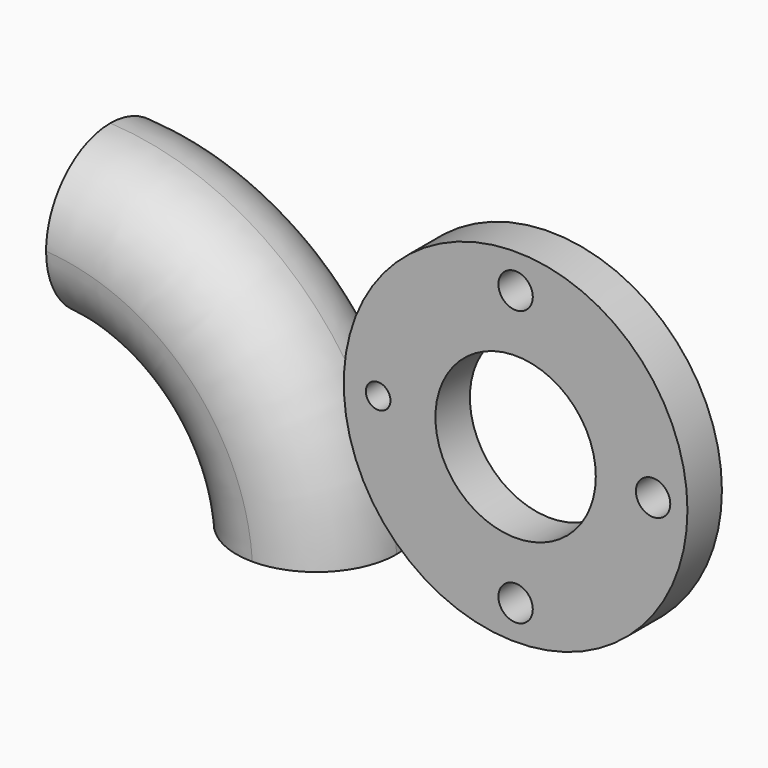
from build123d import *

# Parameters (mm, degrees)
F1_DEPTH    = 44.45
F2_T2_ANGLE = 160.6979741432
F2_T4_ANGLE = 241.2853924859
F2_T6_ANGLE = 160.6979741432
F2_T8_ANGLE = 241.2853924859
F3_R        = 95.25
F3_R_2      = 9.525
F3_R_3      = 6.8244070411
F3_R_4      = 44.45
F4_DEPTH    = 23.876


# Not quite as in the source:
# - a fillet or chamfer that OpenCascade refuses, or shapes differently, is made with other operations: its cross-section is extruded or revolved along the edge and cut away or added


with BuildPart() as f1:
    # F0 (on Front) → F1 (new body, symmetric)
    with BuildSketch(Plane.XZ):
        with BuildLine():
            Line((-141.7071309926, 88.9), (-141.7071309926, 0))
            ThreePointArc((-141.7071309926, 0), (-94.3529466908, -22.4958156982), (-71.8571309926, -69.85))
            Line((-71.8571309926, -69.85), (-27.4071309926, -69.85))
            Line((-27.4071309926, -69.85), (17.0428690074, -69.85))
            ThreePointArc((17.0428690074, -69.85), (-31.6875363662, 40.1695946264), (-141.7071309926, 88.9))
        make_face()
    extrude(amount=F1_DEPTH, both=True)

    # F2: fillet of radius 44.45 on 4 edges, made by hand

    # F2_s1 → F2_t2 (revolve, cut)
    with BuildSketch(Plane(origin=(-86.9289094925, 0, -122.5517924567), x_dir=(0, 1, 0), z_dir=(-0.5785551991, 0, -0.8156432318))):
        with BuildLine():
            ThreePointArc((0, 89.9560683749), (-31.4308964237, 76.9369647986), (-44.45, 45.5060683749))
            Line((-44.45, 45.5060683749), (-44.45, 89.9560683749))
            Line((-44.45, 89.9560683749), (0, 89.9560683749))
        make_face()
    revolve(axis=Axis((-149.8075815664, -44.45, -77.9504505738), (0, -1, 0)), revolution_arc=F2_T2_ANGLE, mode=Mode.SUBTRACT)

    # F2_s3 → F2_t4 (revolve, cut)
    with BuildSketch(Plane(origin=(-27.8850809272, 0, -108.9421849099), x_dir=(0, 1, 0), z_dir=(-0.2479680397, 0, -0.9687682134))):
        with BuildLine():
            ThreePointArc((-44.45, -248.3074320129), (-31.4308964237, -216.8765355892), (0, -203.8574320129))
            Line((0, -203.8574320129), (-44.45, -203.8574320129))
            Line((-44.45, -203.8574320129), (-44.45, -248.3074320129))
        make_face()
    revolve(axis=Axis((-149.6357477999, -44.45, -77.7786168073), (0, 1, 0)), revolution_arc=F2_T4_ANGLE, mode=Mode.SUBTRACT)

    # F2_s5 → F2_t6 (revolve, cut)
    with BuildSketch(Plane(origin=(-86.9289094925, 0, -122.5517924567), x_dir=(0, 1, 0), z_dir=(-0.5785551991, 0, -0.8156432318))):
        with BuildLine():
            ThreePointArc((0, 89.9560683749), (31.4308964237, 76.9369647986), (44.45, 45.5060683749))
            Line((44.45, 45.5060683749), (44.45, 89.9560683749))
            Line((44.45, 89.9560683749), (0, 89.9560683749))
        make_face()
    revolve(axis=Axis((-149.8075815664, 44.45, -77.9504505738), (0, -1, 0)), revolution_arc=F2_T6_ANGLE, mode=Mode.SUBTRACT)

    # F2_s7 → F2_t8 (revolve, cut)
    with BuildSketch(Plane(origin=(-27.8850809272, 0, -108.9421849099), x_dir=(0, 1, 0), z_dir=(-0.2479680397, 0, -0.9687682134))):
        with BuildLine():
            ThreePointArc((0, -203.8574320129), (31.4308964237, -216.8765355892), (44.45, -248.3074320129))
            Line((44.45, -248.3074320129), (44.45, -203.8574320129))
            Line((44.45, -203.8574320129), (0, -203.8574320129))
        make_face()
    revolve(axis=Axis((-149.6357477999, 44.45, -77.7786168073), (0, 1, 0)), revolution_arc=F2_T8_ANGLE, mode=Mode.SUBTRACT)


with BuildPart() as f4:
    # F3 (on Front) → F4 (new body)
    with BuildSketch(Plane.XZ):
        with Locations((102.0744070411, 19.9546236545)):
            Circle(F3_R)
        with Locations((102.0744070411, -56.2453763455)):
            Circle(F3_R_2, mode=Mode.SUBTRACT)
        with Locations((25.8744070411, 19.9546236545)):
            Circle(F3_R_3, mode=Mode.SUBTRACT)
        with Locations((102.0744070411, 19.9546236545)):
            Circle(F3_R_4, mode=Mode.SUBTRACT)
        with Locations((178.2744070411, 19.9546236545)):
            Circle(F3_R_2, mode=Mode.SUBTRACT)
        with Locations((102.0744070411, 96.1546236545)):
            Circle(F3_R_2, mode=Mode.SUBTRACT)
    extrude(amount=F4_DEPTH)


solid = Compound([f1.part, f4.part])
